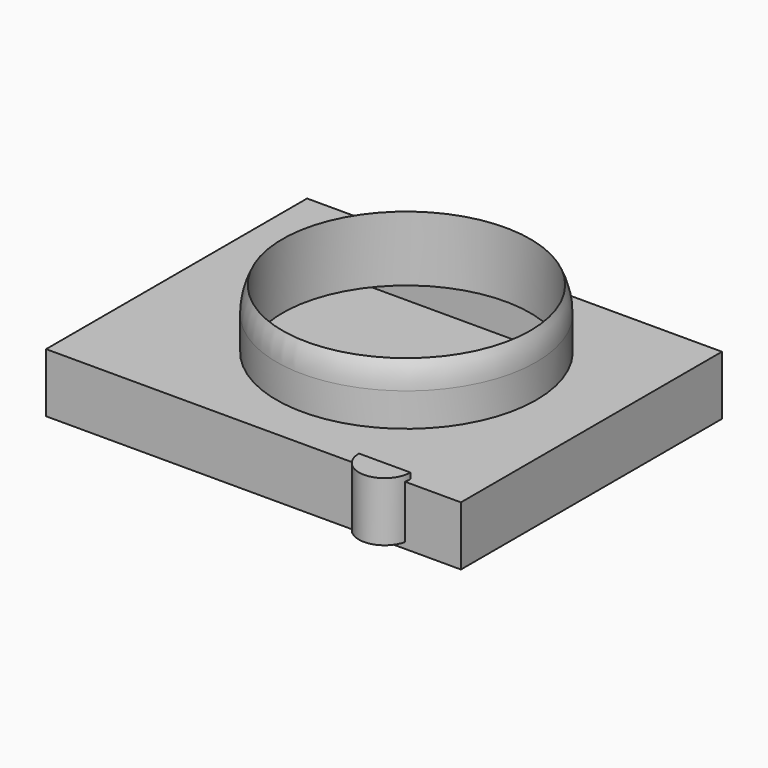
from build123d import *

# Parameters (mm, degrees)
F0_W     = 178.1788319349
F0_H     = 140.1249915361
F1_DEPTH = 25.4
F2_R     = 55.7882871659
F3_DEPTH = 25.4
F4_T     = -2.54
F7_DEPTH = 25.4


# Not quite as in the source:
# - a fillet or chamfer that OpenCascade refuses, or shapes differently, is made with other operations: its cross-section is extruded or revolved along the edge and cut away or added


with BuildPart() as f1:
    # F0 (on Top) → F1 (new body)
    with BuildSketch(Plane.XY):
        with Locations((89.0894159675, 70.0624957681)):
            Rectangle(F0_W, F0_H)
    extrude(amount=F1_DEPTH)

    # F2 (on face) → F3 (join)
    with BuildSketch(Plane.XY.offset(25.4)):
        with Locations((95.6915691495, 73.8431587815)):
            Circle(F2_R)
    extrude(amount=F3_DEPTH)

    # F4
    f4_openings = [f1.faces().sort_by_distance(p)[0] for p in [
        (95.691569, 73.843159, 50.8),
    ]]
    offset(amount=F4_T, openings=f4_openings, kind=Kind.INTERSECTION)

    # F5: fillet of radius 25.4 on 1 edges, made by hand

    # F5_s1 → F5_t2 (revolve, cut)
    with BuildSketch(Plane.XZ.offset(-73.8431587815)):
        with BuildLine():
            ThreePointArc((151.4798563154, 39.7283966834), (150.8367139512, 45.4080093463), (148.9398563154, 50.8))
            Line((148.9398563154, 50.8), (151.4798563154, 50.8))
            Line((151.4798563154, 50.8), (151.4798563154, 39.7283966834))
        make_face()
    revolve(axis=Axis((95.6915691495, 73.8431587815, 50.8), (0, 0, 1)), mode=Mode.SUBTRACT)

    # F6 (on face) → F7 (join)
    with BuildSketch(Plane.XY.offset(2.54)):
        with BuildLine():
            ThreePointArc((132.352274685, 2.54), (143.3852910995, -8.4930164146), (154.4183075141, 2.54))
            Line((154.4183075141, 2.54), (132.352274685, 2.54))
        make_face()
    extrude(amount=F7_DEPTH)


solid = f1.part
